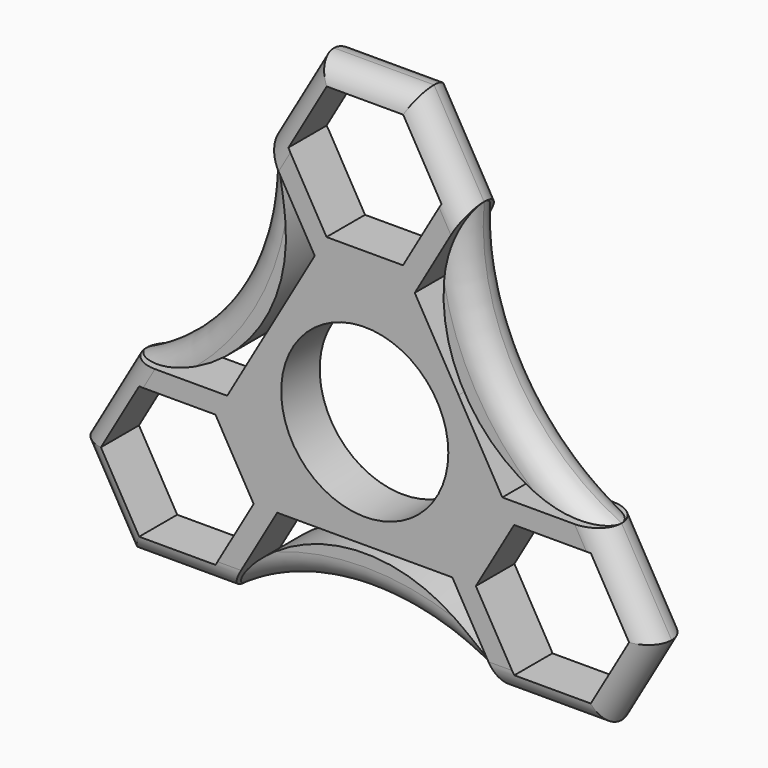
from build123d import *

# Parameters (mm, degrees)
F1_DEPTH      = 6.35
F0_R          = 11.0236
F2_T1_DEPTH   = 29.0732271537
F2_T3_DEPTH   = 29.0732271537
F2_T5_DEPTH   = 29.0732271537
F2_T7_DEPTH   = 29.0732271537
F2_T9_DEPTH   = 29.0732271537
F2_T11_DEPTH  = 29.0732271537
F2_T13_DEPTH  = 29.0732271537
F2_T15_DEPTH  = 29.0732271537
F2_T17_DEPTH  = 29.0732271537
F2_2_T2_ANGLE = 98.3752988321
F2_3_T2_ANGLE = 98.3752988321
F2_4_T2_ANGLE = 98.3752988321
F3_T1_DEPTH   = 29.0732271537
F3_T3_DEPTH   = 29.0732271537
F3_T5_DEPTH   = 29.0732271537
F3_T7_DEPTH   = 29.0732271537
F3_T9_DEPTH   = 29.0732271537
F3_T11_DEPTH  = 29.0732271537
F3_T13_DEPTH  = 29.0732271537
F3_T15_DEPTH  = 29.0732271537
F3_T17_DEPTH  = 29.0732271537
F3_2_T2_ANGLE = 98.3752988321
F3_3_T2_ANGLE = 98.3752988321
F3_4_T2_ANGLE = 98.3752988321


# Not quite as in the source:
# - a fillet or chamfer that OpenCascade refuses, or shapes differently, is made with other operations: its cross-section is extruded or revolved along the edge and cut away or added


with BuildPart() as f1:
    # F0 (on Front) → F1 (new body)
    with BuildSketch(Plane.XZ):
        with BuildLine():
            ThreePointArc((-31.34578949, -2.8575), (-13.1982271537, 7.62), (-13.1982271537, 28.575))
            ThreePointArc((-13.1982271537, 28.575), (-17.3377575298, 10.009958977), (-31.34578949, -2.8575))
        make_face()
    extrude(amount=F1_DEPTH)

    # F2#2: fillet of radius 3.175 on 1 edges, made by hand

    # F2_2_s1 → F2_2_t2 (revolve, cut)
    with BuildSketch(Plane(origin=(-12.8777682078, 0, 37.0055953838), x_dir=(0, 1, 0), z_dir=(-0.3286630709, 0, 0.9444472382))):
        with BuildLine():
            ThreePointArc((-3.175, 2.0859779117), (-5.4200640303, 1.156041942), (-6.35, -1.0890220883))
            Line((-6.35, -1.0890220883), (-6.35, 2.0859779117))
            Line((-6.35, 2.0859779117), (-3.175, 2.0859779117))
        make_face()
    revolve(axis=Axis((-44.8340641, -6.35, 25.884958977), (0, 1, 0)), revolution_arc=F2_2_T2_ANGLE, mode=Mode.SUBTRACT)

    # F3#4: fillet of radius 3.175 on 1 edges, made by hand

    # F3_4_s1 → F3_4_t2 (revolve, cut)
    with BuildSketch(Plane(origin=(-12.8777682078, 0, 37.0055953838), x_dir=(0, 1, 0), z_dir=(-0.3286630709, 0, 0.9444472382))):
        with BuildLine():
            ThreePointArc((-3.175, 2.0859779117), (-0.9299359697, 1.156041942), (0, -1.0890220883))
            Line((0, -1.0890220883), (0, 2.0859779117))
            Line((0, 2.0859779117), (-3.175, 2.0859779117))
        make_face()
    revolve(axis=Axis((-44.8340641, 0, 25.884958977), (0, 1, 0)), revolution_arc=F3_4_T2_ANGLE, mode=Mode.SUBTRACT)


with BuildPart() as f1b:
    # F0 (on Front) → F1, piece 2 (new body)
    with BuildSketch(Plane.XZ):
        with BuildLine():
            ThreePointArc((13.1982271537, 28.575), (13.1982271537, 7.62), (31.34578949, -2.8575))
            ThreePointArc((31.34578949, -2.8575), (17.3377575298, 10.009958977), (13.1982271537, 28.575))
        make_face()
    extrude(amount=F1_DEPTH)

    # F2#4: fillet of radius 3.175 on 1 edges, made by hand

    # F2_4_s1 → F2_4_t2 (revolve, cut)
    with BuildSketch(Plane(origin=(38.4866697884, 0, -7.3503232799), x_dir=(0, 1, 0), z_dir=(0.9822468363, 0, -0.1875930505))):
        with BuildLine():
            ThreePointArc((-3.175, 2.0859779117), (-5.4200640303, 1.156041942), (-6.35, -1.0890220883))
            Line((-6.35, -1.0890220883), (-6.35, 2.0859779117))
            Line((-6.35, 2.0859779117), (-3.175, 2.0859779117))
        make_face()
    revolve(axis=Axis((44.8340641, -6.35, 25.884958977), (0, 1, 0)), revolution_arc=F2_4_T2_ANGLE, mode=Mode.SUBTRACT)

    # F3#2: fillet of radius 3.175 on 1 edges, made by hand

    # F3_2_s1 → F3_2_t2 (revolve, cut)
    with BuildSketch(Plane(origin=(38.4866697884, 0, -7.3503232799), x_dir=(0, 1, 0), z_dir=(0.9822468363, 0, -0.1875930505))):
        with BuildLine():
            ThreePointArc((-3.175, 2.0859779117), (-0.9299359697, 1.156041942), (0, -1.0890220883))
            Line((0, -1.0890220883), (0, 2.0859779117))
            Line((0, 2.0859779117), (-3.175, 2.0859779117))
        make_face()
    revolve(axis=Axis((44.8340641, 0, 25.884958977), (0, 1, 0)), revolution_arc=F3_2_T2_ANGLE, mode=Mode.SUBTRACT)


with BuildPart() as f1c:
    # F0 (on Front) → F1, piece 3 (new body)
    with BuildSketch(Plane.XZ):
        with BuildLine():
            ThreePointArc((18.1475623363, -25.7175), (0, -15.24), (-18.1475623363, -25.7175))
            ThreePointArc((-18.1475623363, -25.7175), (0, -20.019917954), (18.1475623363, -25.7175))
        make_face()
    extrude(amount=F1_DEPTH)

    # F2#3: fillet of radius 3.175 on 1 edges, made by hand

    # F2_3_s1 → F2_3_t2 (revolve, cut)
    with BuildSketch(Plane(origin=(-25.6089015806, 0, -29.6552721039), x_dir=(0, 1, 0), z_dir=(-0.6535837654, 0, -0.7568541878))):
        with BuildLine():
            ThreePointArc((-3.175, 2.0859779117), (-5.4200640303, 1.156041942), (-6.35, -1.0890220883))
            Line((-6.35, -1.0890220883), (-6.35, 2.0859779117))
            Line((-6.35, 2.0859779117), (-3.175, 2.0859779117))
        make_face()
    revolve(axis=Axis((0, -6.35, -51.769917954), (0, 1, 0)), revolution_arc=F2_3_T2_ANGLE, mode=Mode.SUBTRACT)

    # F3#3: fillet of radius 3.175 on 1 edges, made by hand

    # F3_3_s1 → F3_3_t2 (revolve, cut)
    with BuildSketch(Plane(origin=(-25.6089015806, 0, -29.6552721039), x_dir=(0, 1, 0), z_dir=(-0.6535837654, 0, -0.7568541878))):
        with BuildLine():
            ThreePointArc((-3.175, 2.0859779117), (-0.9299359697, 1.156041942), (0, -1.0890220883))
            Line((0, -1.0890220883), (0, 2.0859779117))
            Line((0, 2.0859779117), (-3.175, 2.0859779117))
        make_face()
    revolve(axis=Axis((0, 0, -51.769917954), (0, 1, 0)), revolution_arc=F3_3_T2_ANGLE, mode=Mode.SUBTRACT)


with BuildPart() as f1d:
    # F0 (on Front) → F1, piece 4 (new body)
    with BuildSketch(Plane.XZ):
        Polygon((-6.5991135768, 17.145), (6.5991135768, 17.145), (13.1982271537, 28.575), (6.5991135768, 40.005), (-6.5991135768, 40.005), (-13.1982271537, 28.575), align=None)
        Polygon((10.0893114241, 28.575), (5.0446557121, 19.8374), (-5.0446557121, 19.8374), (-10.0893114241, 28.575), (-5.0446557121, 37.3126), (5.0446557121, 37.3126), align=None, mode=Mode.SUBTRACT)
        Polygon((-18.1475623363, -25.7175), (-11.5484487595, -14.2875), (-18.1475623363, -2.8575), (-31.34578949, -2.8575), (-37.9449030668, -14.2875), (-31.34578949, -25.7175), align=None)
        Polygon((-14.657364489, -14.2875), (-19.7020202011, -23.0251), (-29.7913316252, -23.0251), (-34.8359873373, -14.2875), (-29.7913316252, -5.5499), (-19.7020202011, -5.5499), align=None, mode=Mode.SUBTRACT)
        Polygon((31.34578949, -2.8575), (18.1475623363, -2.8575), (11.5484487595, -14.2875), (18.1475623363, -25.7175), (31.34578949, -25.7175), (37.9449030668, -14.2875), align=None)
        Polygon((19.7020202011, -5.5499), (29.7913316252, -5.5499), (34.8359873373, -14.2875), (29.7913316252, -23.0251), (19.7020202011, -23.0251), (14.657364489, -14.2875), align=None, mode=Mode.SUBTRACT)
        with BuildLine():
            ThreePointArc((0, -14.2875), (10.1027881362, -10.1027881362), (14.2875, 0))
            ThreePointArc((14.2875, 0), (13.8006654478, 3.6978763431), (12.3733387473, 7.1437486304))
            ThreePointArc((12.3733387473, 7.1437486304), (5.17e-08, 14.2875), (-12.3733386957, 7.1437487198))
            ThreePointArc((-12.3733386957, 7.1437487198), (-12.373337587, -7.1437506401), (0, -14.2875))
        make_face()
        Circle(F0_R, mode=Mode.SUBTRACT)
        with BuildLine():
            ThreePointArc((12.3733387473, 7.1437486304), (13.8006654478, 3.6978763431), (14.2875, 0))
            ThreePointArc((14.2875, 0), (10.1027881362, -10.1027881362), (0, -14.2875))
            Line((0, -14.2875), (11.5484487595, -14.2875))
            Line((11.5484487595, -14.2875), (18.1475623363, -2.8575))
            Line((18.1475623363, -2.8575), (12.3733387473, 7.1437486304))
        make_face()
        with BuildLine():
            Line((-11.5484487595, -14.2875), (0, -14.2875))
            ThreePointArc((0, -14.2875), (-12.373337587, -7.1437506401), (-12.3733386957, 7.1437487198))
            Line((-12.3733386957, 7.1437487198), (-18.1475623363, -2.8575))
            Line((-18.1475623363, -2.8575), (-11.5484487595, -14.2875))
        make_face()
        with BuildLine():
            ThreePointArc((-12.3733386957, 7.1437487198), (5.17e-08, 14.2875), (12.3733387473, 7.1437486304))
            Line((12.3733387473, 7.1437486304), (6.5991135768, 17.145))
            Line((6.5991135768, 17.145), (-6.5991135768, 17.145))
            Line((-6.5991135768, 17.145), (-12.3733386957, 7.1437487198))
        make_face()
    extrude(amount=F1_DEPTH)

    # F2: fillet of radius 3.175 on 9 edges, made by hand

    # F2_s2 → F2_t1 (cut)
    with BuildSketch(Plane(origin=(19.641644745, 0, 34.0203266425), x_dir=(0, 1, 0), z_dir=(-0.5, 0, -0.8660254038))):
        with BuildLine():
            ThreePointArc((-3.175, -25.7175), (-5.4200640303, -24.7875640303), (-6.35, -22.5425))
            Line((-6.35, -22.5425), (-6.35, -25.7175))
            Line((-6.35, -25.7175), (-3.175, -25.7175))
        make_face()
    extrude(amount=F2_T1_DEPTH, mode=Mode.SUBTRACT)

    # F2_s4 → F2_t3 (cut)
    with BuildSketch(Plane.YZ.offset(-14.5366135768)):
        with BuildLine():
            ThreePointArc((-3.175, 40.005), (-5.4200640303, 39.0750640303), (-6.35, 36.83))
            Line((-6.35, 36.83), (-6.35, 40.005))
            Line((-6.35, 40.005), (-3.175, 40.005))
        make_face()
    extrude(amount=F2_T3_DEPTH, mode=Mode.SUBTRACT)

    # F2_s6 → F2_t5 (cut)
    with BuildSketch(Plane(origin=(-5.1050311682, 0, 8.8421733575), x_dir=(0, 1, 0), z_dir=(-0.5, 0, 0.8660254038))):
        with BuildLine():
            ThreePointArc((-3.175, -25.7175), (-5.4200640303, -24.7875640303), (-6.35, -22.5425))
            Line((-6.35, -22.5425), (-6.35, -25.7175))
            Line((-6.35, -25.7175), (-3.175, -25.7175))
        make_face()
    extrude(amount=F2_T5_DEPTH, mode=Mode.SUBTRACT)

    # F2_s8 → F2_t7 (cut)
    with BuildSketch(Plane(origin=(-5.1050311682, 0, -8.8421733575), x_dir=(0, 1, 0), z_dir=(-0.5, 0, -0.8660254038))):
        with BuildLine():
            ThreePointArc((-3.175, -25.7175), (-5.4200640303, -24.7875640303), (-6.35, -22.5425))
            Line((-6.35, -22.5425), (-6.35, -25.7175))
            Line((-6.35, -25.7175), (-3.175, -25.7175))
        make_face()
    extrude(amount=F2_T7_DEPTH, mode=Mode.SUBTRACT)

    # F2_s10 → F2_t9 (cut)
    with BuildSketch(Plane(origin=(-7.2683067884, 0, 12.5890766425), x_dir=(0, 1, 0), z_dir=(0.5, 0, -0.8660254038))):
        with BuildLine():
            ThreePointArc((-3.175, -40.005), (-5.4200640303, -39.0750640303), (-6.35, -36.83))
            Line((-6.35, -36.83), (-6.35, -40.005))
            Line((-6.35, -40.005), (-3.175, -40.005))
        make_face()
    extrude(amount=F2_T9_DEPTH, mode=Mode.SUBTRACT)

    # F2_s12 → F2_t11 (cut)
    with BuildSketch(Plane.YZ.offset(-39.28328949)):
        with BuildLine():
            ThreePointArc((-3.175, -25.7175), (-5.4200640303, -24.7875640303), (-6.35, -22.5425))
            Line((-6.35, -22.5425), (-6.35, -25.7175))
            Line((-6.35, -25.7175), (-3.175, -25.7175))
        make_face()
    extrude(amount=F2_T11_DEPTH, mode=Mode.SUBTRACT)

    # F2_s14 → F2_t13 (cut)
    with BuildSketch(Plane.YZ.offset(10.2100623363)):
        with BuildLine():
            ThreePointArc((-3.175, -25.7175), (-5.4200640303, -24.7875640303), (-6.35, -22.5425))
            Line((-6.35, -22.5425), (-6.35, -25.7175))
            Line((-6.35, -25.7175), (-3.175, -25.7175))
        make_face()
    extrude(amount=F2_T13_DEPTH, mode=Mode.SUBTRACT)

    # F2_s16 → F2_t15 (cut)
    with BuildSketch(Plane(origin=(-7.2683067884, 0, -12.5890766425), x_dir=(0, 1, 0), z_dir=(0.5, 0, 0.8660254038))):
        with BuildLine():
            ThreePointArc((-3.175, -40.005), (-5.4200640303, -39.0750640303), (-6.35, -36.83))
            Line((-6.35, -36.83), (-6.35, -40.005))
            Line((-6.35, -40.005), (-3.175, -40.005))
        make_face()
    extrude(amount=F2_T15_DEPTH, mode=Mode.SUBTRACT)

    # F2_s18 → F2_t17 (cut)
    with BuildSketch(Plane(origin=(19.641644745, 0, -34.0203266425), x_dir=(0, 1, 0), z_dir=(-0.5, 0, 0.8660254038))):
        with BuildLine():
            ThreePointArc((-3.175, -25.7175), (-5.4200640303, -24.7875640303), (-6.35, -22.5425))
            Line((-6.35, -22.5425), (-6.35, -25.7175))
            Line((-6.35, -25.7175), (-3.175, -25.7175))
        make_face()
    extrude(amount=F2_T17_DEPTH, mode=Mode.SUBTRACT)

    # F3: fillet of radius 3.175 on 9 edges, made by hand

    # F3_s2 → F3_t1 (cut)
    with BuildSketch(Plane.YZ.offset(-14.5366135768)):
        with BuildLine():
            ThreePointArc((0, 36.83), (-0.9299359697, 39.0750640303), (-3.175, 40.005))
            Line((-3.175, 40.005), (0, 40.005))
            Line((0, 40.005), (0, 36.83))
        make_face()
    extrude(amount=F3_T1_DEPTH, mode=Mode.SUBTRACT)

    # F3_s4 → F3_t3 (cut)
    with BuildSketch(Plane(origin=(-5.1050311682, 0, 8.8421733575), x_dir=(0, 1, 0), z_dir=(-0.5, 0, 0.8660254038))):
        with BuildLine():
            ThreePointArc((0, -22.5425), (-0.9299359697, -24.7875640303), (-3.175, -25.7175))
            Line((-3.175, -25.7175), (0, -25.7175))
            Line((0, -25.7175), (0, -22.5425))
        make_face()
    extrude(amount=F3_T3_DEPTH, mode=Mode.SUBTRACT)

    # F3_s6 → F3_t5 (cut)
    with BuildSketch(Plane(origin=(19.641644745, 0, -34.0203266425), x_dir=(0, 1, 0), z_dir=(-0.5, 0, 0.8660254038))):
        with BuildLine():
            ThreePointArc((0, -22.5425), (-0.9299359697, -24.7875640303), (-3.175, -25.7175))
            Line((-3.175, -25.7175), (0, -25.7175))
            Line((0, -25.7175), (0, -22.5425))
        make_face()
    extrude(amount=F3_T5_DEPTH, mode=Mode.SUBTRACT)

    # F3_s8 → F3_t7 (cut)
    with BuildSketch(Plane(origin=(-7.2683067884, 0, -12.5890766425), x_dir=(0, 1, 0), z_dir=(0.5, 0, 0.8660254038))):
        with BuildLine():
            ThreePointArc((0, -36.83), (-0.9299359697, -39.0750640303), (-3.175, -40.005))
            Line((-3.175, -40.005), (0, -40.005))
            Line((0, -40.005), (0, -36.83))
        make_face()
    extrude(amount=F3_T7_DEPTH, mode=Mode.SUBTRACT)

    # F3_s10 → F3_t9 (cut)
    with BuildSketch(Plane.YZ.offset(10.2100623363)):
        with BuildLine():
            ThreePointArc((0, -22.5425), (-0.9299359697, -24.7875640303), (-3.175, -25.7175))
            Line((-3.175, -25.7175), (0, -25.7175))
            Line((0, -25.7175), (0, -22.5425))
        make_face()
    extrude(amount=F3_T9_DEPTH, mode=Mode.SUBTRACT)

    # F3_s12 → F3_t11 (cut)
    with BuildSketch(Plane.YZ.offset(-39.28328949)):
        with BuildLine():
            ThreePointArc((0, -22.5425), (-0.9299359697, -24.7875640303), (-3.175, -25.7175))
            Line((-3.175, -25.7175), (0, -25.7175))
            Line((0, -25.7175), (0, -22.5425))
        make_face()
    extrude(amount=F3_T11_DEPTH, mode=Mode.SUBTRACT)

    # F3_s14 → F3_t13 (cut)
    with BuildSketch(Plane(origin=(-7.2683067884, 0, 12.5890766425), x_dir=(0, 1, 0), z_dir=(0.5, 0, -0.8660254038))):
        with BuildLine():
            ThreePointArc((0, -36.83), (-0.9299359697, -39.0750640303), (-3.175, -40.005))
            Line((-3.175, -40.005), (0, -40.005))
            Line((0, -40.005), (0, -36.83))
        make_face()
    extrude(amount=F3_T13_DEPTH, mode=Mode.SUBTRACT)

    # F3_s16 → F3_t15 (cut)
    with BuildSketch(Plane(origin=(-5.1050311682, 0, -8.8421733575), x_dir=(0, 1, 0), z_dir=(-0.5, 0, -0.8660254038))):
        with BuildLine():
            ThreePointArc((0, -22.5425), (-0.9299359697, -24.7875640303), (-3.175, -25.7175))
            Line((-3.175, -25.7175), (0, -25.7175))
            Line((0, -25.7175), (0, -22.5425))
        make_face()
    extrude(amount=F3_T15_DEPTH, mode=Mode.SUBTRACT)

    # F3_s18 → F3_t17 (cut)
    with BuildSketch(Plane(origin=(19.641644745, 0, 34.0203266425), x_dir=(0, 1, 0), z_dir=(-0.5, 0, -0.8660254038))):
        with BuildLine():
            ThreePointArc((0, -22.5425), (-0.9299359697, -24.7875640303), (-3.175, -25.7175))
            Line((-3.175, -25.7175), (0, -25.7175))
            Line((0, -25.7175), (0, -22.5425))
        make_face()
    extrude(amount=F3_T17_DEPTH, mode=Mode.SUBTRACT)


solid = Compound([f1.part, f1b.part, f1c.part, f1d.part])
